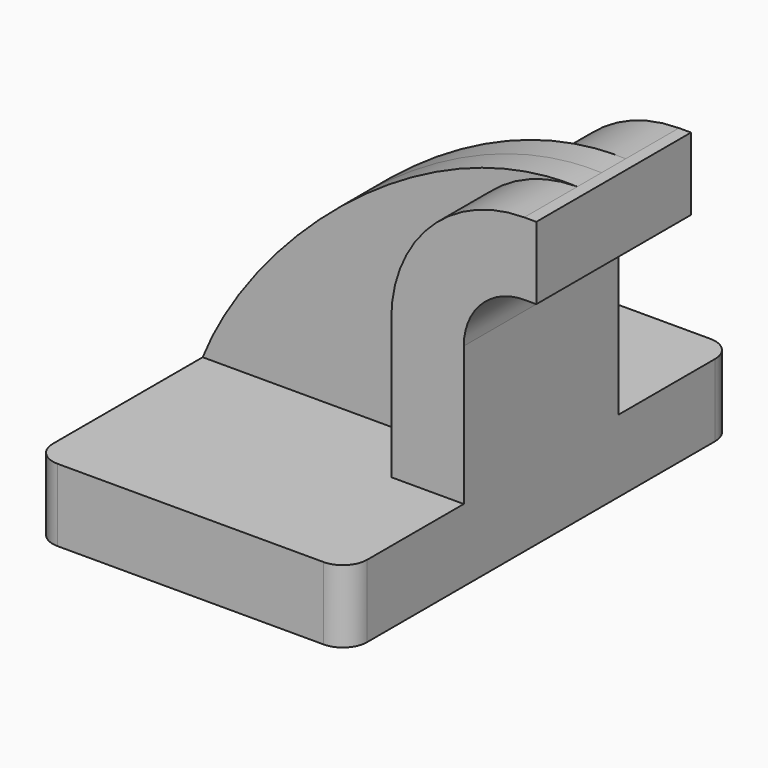
from build123d import *

# Parameters (mm, degrees)
F1_DEPTH = 63.5
F2_DEPTH = 25.4
F3_DEPTH = 7.9375
F5_R     = 6.35


# Not quite as in the source:
# - the program builds the solid bodies; features that only make, move or delete a surface that nothing else refers to are left out


with BuildPart() as f1:
    # F0 (on Front) → F1 (new body, symmetric)
    with BuildSketch(Plane.XZ):
        Polygon((22.225, 9.525), (-41.275, 9.525), (-41.275, -9.525), (41.275, -9.525), (41.275, 9.525), align=None)
    extrude(amount=F1_DEPTH, both=True)

    # F0 (on Front) → F2 (join, symmetric)
    with BuildSketch(Plane.XZ):
        with BuildLine():
            Line((22.225, 46.0502), (22.225, 9.525))
            Line((22.225, 9.525), (41.275, 9.525))
            Line((41.275, 9.525), (41.275, 46.0502))
            ThreePointArc((41.275, 46.0502), (45.9246798487, 57.2755201513), (57.15, 61.9252))
            Line((57.15, 61.9252), (60.325, 61.9252))
            Line((60.325, 61.9252), (60.325, 80.9752))
            Line((60.325, 80.9752), (57.15, 80.9752))
            ThreePointArc((57.15, 80.9752), (32.4542956671, 70.7459043329), (22.225, 46.0502))
        make_face()
    extrude(amount=F2_DEPTH, both=True)

    # F0 (on Front) → F3 (join, symmetric)
    with BuildSketch(Plane.XZ):
        with BuildLine():
            add(Edge.make_bspline(
                [(-41.275, 9.525), (-28.4558665007, 41.9093370438), (15.8414896578, 82.5819298625), (57.15, 80.9752)],
                knots=[0, 0, 0, 0, 121.6248811101, 121.6248811101, 121.6248811101, 121.6248811101], degree=3))
            Line((-41.275, 9.525), (22.225, 9.525))
            Line((22.225, 9.525), (22.225, 46.0502))
            ThreePointArc((22.225, 46.0502), (32.4542956671, 70.7459043329), (57.15, 80.9752))
        make_face()
    extrude(amount=F3_DEPTH, both=True)

    # F5
    f5_edges = [f1.edges().sort_by_distance(p)[0] for p in [
        (-41.275, -63.5, 0),
        (41.275, -63.5, 0),
        (41.275, 63.5, 0),
        (-41.275, 63.5, 0),
    ]]
    fillet(f5_edges, radius=F5_R)


solid = f1.part
